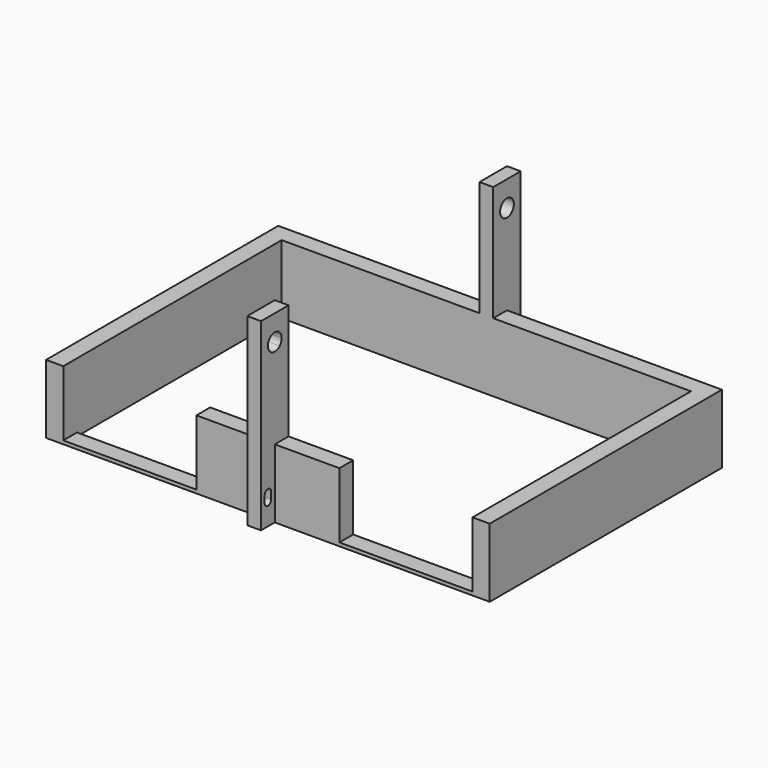
from build123d import *

# Parameters (mm, degrees)
F0_W     = 49.1559793526
F0_H     = 6.35
F0_W_2   = 5.08
F0_W_3   = 23.8690206474
F1_DEPTH = 1.27
F2_DEPTH = 25.4
F3_W     = 5.08
F3_H     = 12.7
F4_DEPTH = 42.624
F6_DEPTH = 25.4
F7_R     = 3.175
F8_DEPTH = 25.4


with BuildPart() as f1:
    # F0 (on Top) → F1 (new body)
    with BuildSketch(Plane.XY):
        with Locations((-50.9870103237, -50.419)):
            Rectangle(F0_W, F0_H)
        Polygon((-75.565, 47.244), (-2.54, 47.244), (-2.54, 53.594), (-81.915, 53.594), (-81.915, -53.594), (-75.565, -53.594), (-75.565, -47.244), align=None)
        with Locations((0, 56.769)):
            Rectangle(F0_W_2, F0_H)
        with Locations((0, 50.419)):
            Rectangle(F0_W_2, F0_H)
        Polygon((2.54, 47.244), (75.565, 47.244), (75.565, -47.244), (75.565, -53.594), (81.915, -53.594), (81.915, 53.594), (2.54, 53.594), align=None)
        with Locations((50.9870103237, -50.419)):
            Rectangle(F0_W, F0_H)
        with Locations((-14.4745103237, -50.419)):
            Rectangle(F0_W_3, F0_H)
        with Locations((0, -50.419)):
            Rectangle(F0_W_2, F0_H)
        with Locations((14.4745103237, -50.419)):
            Rectangle(F0_W_3, F0_H)
        with Locations((0, -56.769)):
            Rectangle(F0_W_2, F0_H)
    extrude(amount=F1_DEPTH)

    # F0 (on Top) → F2 (join)
    with BuildSketch(Plane.XY):
        Polygon((-75.565, 47.244), (-2.54, 47.244), (-2.54, 53.594), (-81.915, 53.594), (-81.915, -53.594), (-75.565, -53.594), (-75.565, -47.244), align=None)
        with Locations((0, 56.769)):
            Rectangle(F0_W_2, F0_H)
        with Locations((0, 50.419)):
            Rectangle(F0_W_2, F0_H)
        Polygon((2.54, 47.244), (75.565, 47.244), (75.565, -47.244), (75.565, -53.594), (81.915, -53.594), (81.915, 53.594), (2.54, 53.594), align=None)
        with Locations((14.4745103237, -50.419)):
            Rectangle(F0_W_3, F0_H)
        with Locations((0, -50.419)):
            Rectangle(F0_W_2, F0_H)
        with Locations((-14.4745103237, -50.419)):
            Rectangle(F0_W_3, F0_H)
        with Locations((0, -56.769)):
            Rectangle(F0_W_2, F0_H)
    extrude(amount=F2_DEPTH)

    # F3 (on face) → F4 (join)
    with BuildSketch(Plane.XY.offset(25.4)):
        Polygon((2.54, 59.944), (-2.54, 59.944), (-2.54, 53.594), (-2.54, 47.244), (2.54, 47.244), (2.54, 53.594), align=None)
        with Locations((0, -53.594)):
            Rectangle(F3_W, F3_H)
    extrude(amount=F4_DEPTH)

    # F5 (on face) → F6 (cut)
    with BuildSketch(Plane.YZ.offset(2.54)):
        with BuildLine():
            Line((-58.2624942683, 8.2038091254), (-58.2624942683, 8.1145596807))
            ThreePointArc((-58.2624942683, 8.1145596807), (-56.7408433733, 6.6593503961), (-55.2631582039, 8.159184403))
            ThreePointArc((-55.2631582039, 8.159184403), (-55.4440615048, 8.8733159724), (-55.9431367352, 9.4151958643))
            ThreePointArc((-55.9431367352, 9.4151958643), (-56.7631582039, 9.1712073255), (-57.5831796726, 9.4151958643))
            ThreePointArc((-57.5831796726, 9.4151958643), (-58.0714851124, 8.8928605581), (-58.2624942683, 8.2038091254))
        make_face()
        with BuildLine():
            ThreePointArc((-58.2624942683, 8.2038091254), (-58.2631582039, 8.159184403), (-58.2624942683, 8.1145596807))
            Line((-58.2624942683, 8.1145596807), (-58.2624942683, 8.2038091254))
        make_face()
        with BuildLine():
            ThreePointArc((-55.9431367352, 9.4151958643), (-55.4440615048, 8.8733159724), (-55.2631582039, 8.159184403))
            Line((-55.2631582039, 8.159184403), (-55.2631582039, 10.6712073255))
            ThreePointArc((-55.2631582039, 10.6712073255), (-55.4440615048, 9.9570757561), (-55.9431367352, 9.4151958643))
        make_face()
        with BuildLine():
            Line((-58.2624942683, 10.6265826032), (-58.2624942683, 8.2038091254))
            ThreePointArc((-58.2624942683, 8.2038091254), (-58.0714851124, 8.8928605581), (-57.5831796726, 9.4151958643))
            ThreePointArc((-57.5831796726, 9.4151958643), (-58.0714851124, 9.9375311705), (-58.2624942683, 10.6265826032))
        make_face()
        with BuildLine():
            ThreePointArc((-57.5831796726, 9.4151958643), (-56.7631582039, 9.659184403), (-55.9431367352, 9.4151958643))
            ThreePointArc((-55.9431367352, 9.4151958643), (-55.4440615048, 9.9570757561), (-55.2631582039, 10.6712073255))
            ThreePointArc((-55.2631582039, 10.6712073255), (-56.7854730345, 12.1710413325), (-58.2624942683, 10.6265826032))
            ThreePointArc((-58.2624942683, 10.6265826032), (-58.0714851124, 9.9375311705), (-57.5831796726, 9.4151958643))
        make_face()
        with BuildLine():
            ThreePointArc((-57.5831796726, 9.4151958643), (-56.7631582039, 9.1712073255), (-55.9431367352, 9.4151958643))
            ThreePointArc((-55.9431367352, 9.4151958643), (-56.7631582039, 9.659184403), (-57.5831796726, 9.4151958643))
        make_face()
    extrude(amount=-F6_DEPTH, mode=Mode.SUBTRACT)

    # F7 (on face) → F8 (cut)
    with BuildSketch(Plane.YZ.offset(2.54)):
        with Locations((53.594, 58.674)):
            Circle(F7_R)
        with BuildLine():
            ThreePointArc((-50.419, 58.674), (-52.3789801022, 61.6073175157), (-55.8390640303, 60.9190640303))
            Line((-55.8390640303, 60.9190640303), (-51.3489359697, 56.4289359697))
            ThreePointArc((-51.3489359697, 56.4289359697), (-50.6606824843, 57.4589801022), (-50.419, 58.674))
        make_face()
        with BuildLine():
            Line((-51.3489359697, 56.4289359697), (-55.8390640303, 60.9190640303))
            ThreePointArc((-55.8390640303, 60.9190640303), (-55.8390640303, 56.4289359697), (-51.3489359697, 56.4289359697))
        make_face()
    extrude(amount=-F8_DEPTH, mode=Mode.SUBTRACT)


solid = f1.part
